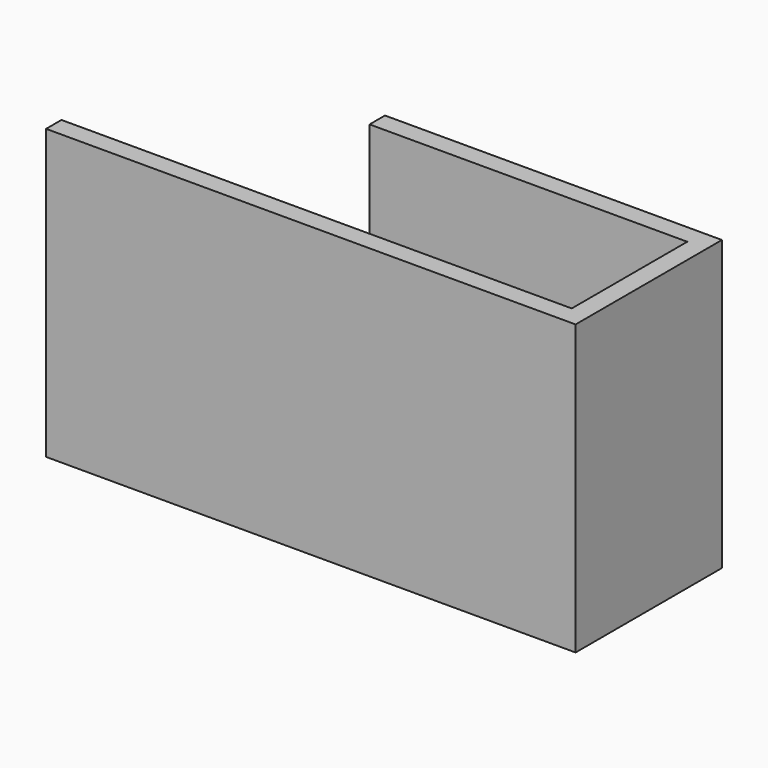
from build123d import *

# Parameters (mm, degrees)
F1_DEPTH = 30


# Not quite as in the source:
# - a feature of the source that left no trace in its solid (it failed there, or was rolled back) is left out


with BuildPart() as f1:
    # F0 (on Top) → F1 (new body)
    with BuildSketch(Plane.XY):
        Polygon((0, 2), (0, 0), (55, 0), (55, 19), (20, 19), (20, 17), (53, 17), (53, 2), align=None)
    extrude(amount=F1_DEPTH)


solid = f1.part
